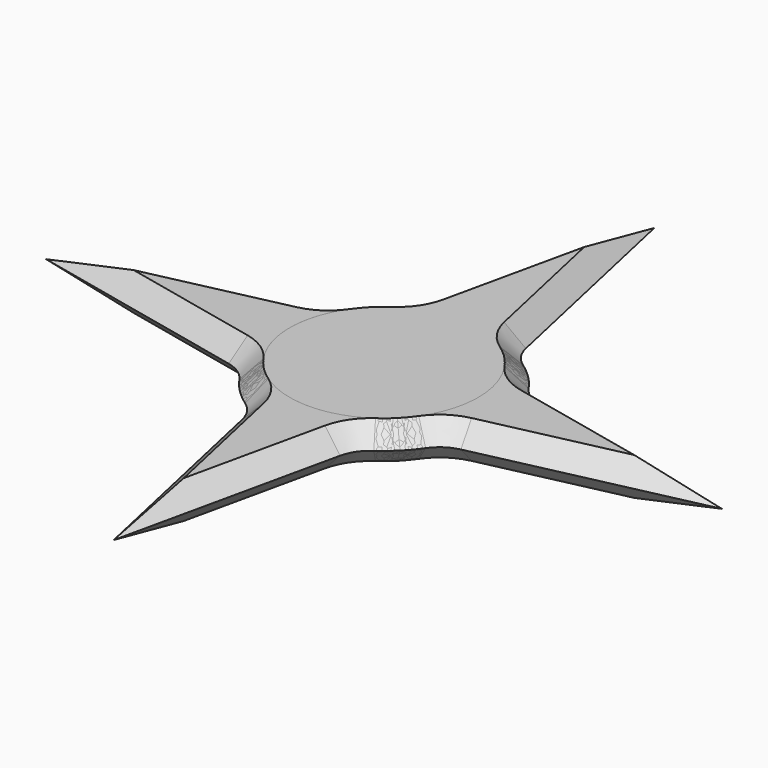
from build123d import *

# Parameters (mm, degrees)
F1_DEPTH  = 3.175
F2_COUNT  = 4
F3_SIZE   = 3.17499
F3_2_SIZE = 3.17499
F3_3_SIZE = 3.17499
F3_4_SIZE = 3.17499


# Not quite as in the source:
# - a fillet or chamfer is up to 0.001 mm smaller than in the source, because OpenCascade refuses the exact size


with BuildPart() as f1:
    # F0 (on Top) → F1 (new body, symmetric)
    with BuildSketch(Plane.XY):
        with BuildLine():
            ThreePointArc((-8.2339935894, 19.5317835541), (-9.164570241, 17.3575820119), (-10.8261973213, 15.6746914343))
            ThreePointArc((-10.8261973213, 15.6746914343), (0, -19.05), (10.8261973213, 15.6746914343))
            ThreePointArc((10.8261973213, 15.6746914343), (9.164570241, 17.3575820119), (8.2339935894, 19.5317835541))
            Line((8.2339935894, 19.5317835541), (0, 56.8605458856))
            Line((0, 56.8605458856), (-8.2339935894, 19.5317835541))
        make_face()
    extrude(amount=F1_DEPTH, both=True)


with BuildPart() as f2_1:
    # F2: instance of F1
    add(f1.part.rotate(Axis((0, 0, 0), (0, 0, 1)), 1 * 360 / F2_COUNT))

    # F3 (size 3.175 in the source; OpenCascade refuses exactly that, so slightly less here)
    f3_edges = [f2_1.edges().sort_by_distance(p)[0] for p in [
        (-38.196165, 4.116997, 3.175),
        (-38.196165, -4.116997, 3.175),
        (-17.357582, -9.16457, 3.175),
        (19.05, 0, 3.175),
        (-17.357582, 9.16457, 3.175),
        (-38.196165, 4.116997, -3.175),
        (-38.196165, -4.116997, -3.175),
        (-17.357582, -9.16457, -3.175),
        (19.05, 0, -3.175),
        (-17.357582, 9.16457, -3.175),
    ]]
    chamfer(f3_edges, length=F3_SIZE)


with BuildPart() as f2_2:
    # F2: instance of F1
    add(f1.part.rotate(Axis((0, 0, 0), (0, 0, 1)), 2 * 360 / F2_COUNT))

    # F3#4 (size 3.175 in the source; OpenCascade refuses exactly that, so slightly less here)
    f3_4_edges = [f2_2.edges().sort_by_distance(p)[0] for p in [
        (-4.116997, -38.196165, 3.175),
        (4.116997, -38.196165, 3.175),
        (9.16457, -17.357582, 3.175),
        (0, 19.05, 3.175),
        (-9.16457, -17.357582, 3.175),
        (-4.116997, -38.196165, -3.175),
        (4.116997, -38.196165, -3.175),
        (9.16457, -17.357582, -3.175),
        (0, 19.05, -3.175),
        (-9.16457, -17.357582, -3.175),
    ]]
    chamfer(f3_4_edges, length=F3_4_SIZE)


with BuildPart() as f2_3:
    # F2: instance of F1
    add(f1.part.rotate(Axis((0, 0, 0), (0, 0, 1)), 3 * 360 / F2_COUNT))

    # F3#3 (size 3.175 in the source; OpenCascade refuses exactly that, so slightly less here)
    f3_3_edges = [f2_3.edges().sort_by_distance(p)[0] for p in [
        (38.196165, -4.116997, 3.175),
        (38.196165, 4.116997, 3.175),
        (17.357582, 9.16457, 3.175),
        (-19.05, 0, 3.175),
        (17.357582, -9.16457, 3.175),
        (38.196165, -4.116997, -3.175),
        (38.196165, 4.116997, -3.175),
        (17.357582, 9.16457, -3.175),
        (-19.05, 0, -3.175),
        (17.357582, -9.16457, -3.175),
    ]]
    chamfer(f3_3_edges, length=F3_3_SIZE)


with BuildPart() as f1_1:
    add(f1.part)

    # F3#2 (size 3.175 in the source; OpenCascade refuses exactly that, so slightly less here)
    f3_2_edges = [f1_1.edges().sort_by_distance(p)[0] for p in [
        (4.116997, 38.196165, 3.175),
        (-4.116997, 38.196165, 3.175),
        (-9.16457, 17.357582, 3.175),
        (0, -19.05, 3.175),
        (9.16457, 17.357582, 3.175),
        (4.116997, 38.196165, -3.175),
        (-4.116997, 38.196165, -3.175),
        (-9.16457, 17.357582, -3.175),
        (0, -19.05, -3.175),
        (9.16457, 17.357582, -3.175),
    ]]
    chamfer(f3_2_edges, length=F3_2_SIZE)


solid = Compound([f2_1.part, f2_2.part, f2_3.part, f1_1.part])
